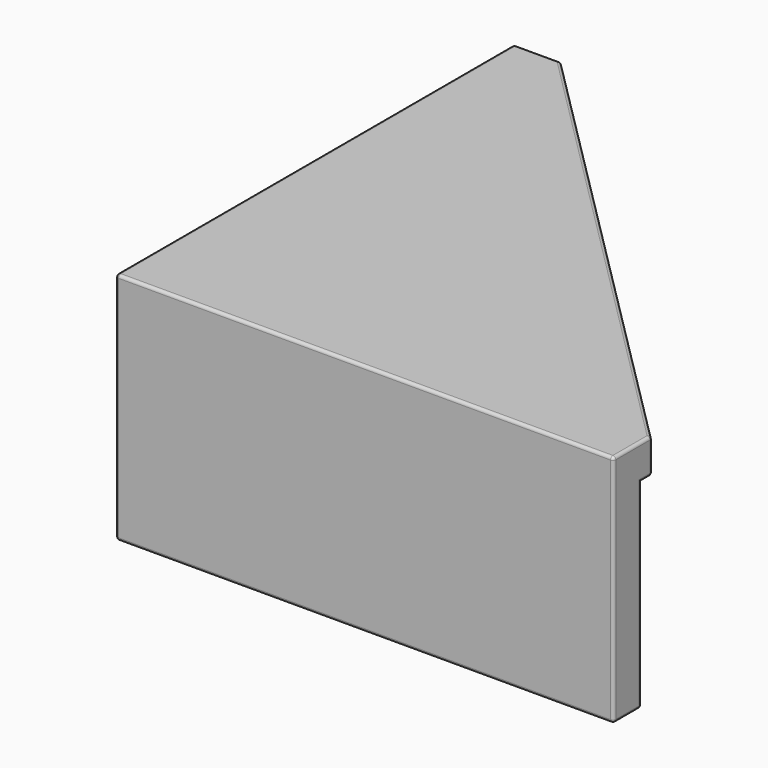
from build123d import *

# Parameters (mm, degrees)
F1_DEPTH = 6
F3_DEPTH = 34
F4_R     = 0.5
F7_DEPTH = 6
F8_R     = 1


# Not quite as in the source:
# - a pattern or mirror of a feature is missing from the dataset's text; its kind, count and spacing are read off the source's solid


with BuildPart() as f1:
    # F0 (on Top) → F1 (new body)
    with BuildSketch(Plane.XY):
        Polygon((0, 85), (0, 0), (85, 0), (85, 8), (8, 85), align=None)
    extrude(amount=F1_DEPTH)

    # F2 (on Top) → F3 (join)
    with BuildSketch(Plane.XY):
        Polygon((0, 85), (0, 0), (85, 0), (85, 6), (6, 6), (6, 85), align=None)
    extrude(amount=-F3_DEPTH)

    # F4
    f4_edges = [f1.edges().sort_by_distance(p)[0] for p in [
        (0, 42.5, -34),
        (42.5, 0, -34),
        (85, 3, -34),
        (45.5, 6, -34),
        (6, 45.5, -34),
        (3, 85, -34),
        (0, 85, -14),
        (0, 42.5, 6),
        (0, 0, -14),
        (8, 85, 3),
        (4, 85, 6),
        (6, 85, -17),
        (7, 85, 0),
        (85, 8, 3),
        (46.5, 46.5, 0),
        (46.5, 46.5, 6),
        (42.5, 0, 6),
        (85, 4, 6),
        (85, 0, -14),
        (85, 7, 0),
        (85, 6, -17),
    ]]
    fillet(f4_edges, radius=F4_R)

    # F6 (on face) → F7 (join)
    with BuildSketch(Plane(origin=(0, 6, 0), x_dir=(-1, 0, 0), z_dir=(0, 1, 0))):
        Polygon((-68, -25.6602540378), (-60.5, -21.3301270189), (-60.5, -12.6698729811), (-68, -8.3397459622), (-75.5, -12.6698729811), (-75.5, -21.3301270189), align=None)
        Polygon((-24, -25.6602540378), (-16.5, -21.3301270189), (-16.5, -12.6698729811), (-24, -8.3397459622), (-31.5, -12.6698729811), (-31.5, -21.3301270189), align=None)
    f7 = extrude(amount=F7_DEPTH)

    # F7_copies: F7 across plane
    add(f7.mirror(Plane(origin=(0, 0, 0), x_dir=(0.7071067812, 0.7071067812, 0), z_dir=(-0.7071067812, 0.7071067812, 0))))

    # F8
    f8_edges = [f1.edges().sort_by_distance(p)[0] for p in [
        (71.75, 12, -23.495191),
        (64.25, 12, -23.495191),
        (60.5, 12, -17),
        (64.25, 12, -10.504809),
        (71.75, 12, -10.504809),
        (75.5, 12, -17),
        (27.75, 12, -23.495191),
        (20.25, 12, -23.495191),
        (16.5, 12, -17),
        (20.25, 12, -10.504809),
        (27.75, 12, -10.504809),
        (31.5, 12, -17),
        (12, 31.5, -17),
        (12, 27.75, -10.504809),
        (12, 20.25, -10.504809),
        (12, 16.5, -17),
        (12, 20.25, -23.495191),
        (12, 27.75, -23.495191),
        (12, 75.5, -17),
        (12, 71.75, -10.504809),
        (12, 64.25, -10.504809),
        (12, 60.5, -17),
        (12, 64.25, -23.495191),
        (12, 71.75, -23.495191),
    ]]
    fillet(f8_edges, radius=F8_R)


solid = f1.part
